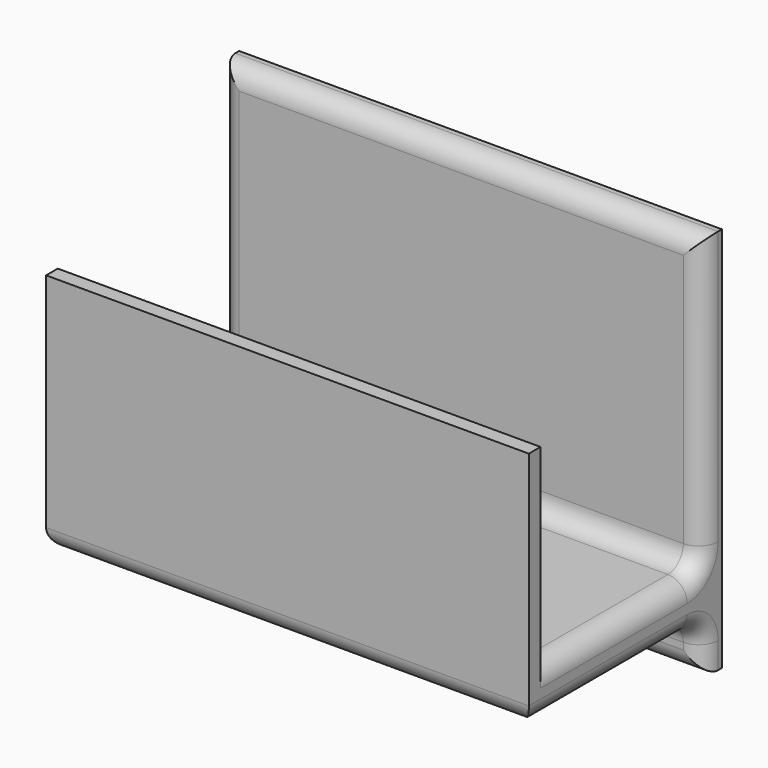
from build123d import *

# Parameters (mm, degrees)
F0_W     = 127
F0_H     = 12.7
F1_DEPTH = 63.5
F0_H_2   = 76.9474954844
F0_H_3   = 11.9525045156
F2_DEPTH = 6.35
F3_W     = 127
F3_H     = 3.8452798724
F4_DEPTH = 50.8
F5_R     = 5.08


with BuildPart() as f1:
    # F0 (on Front) → F1 (new body)
    with BuildSketch(Plane.XZ):
        with Locations((7.5608139634, -7.8621631652)):
            Rectangle(F0_W, F0_H)
    extrude(amount=F1_DEPTH)

    # F0 (on Front) → F2 (join)
    with BuildSketch(Plane.XZ):
        with Locations((7.5608139634, 36.961584577)):
            Rectangle(F0_W, F0_H_2)
        with Locations((7.5608139634, -20.188415423)):
            Rectangle(F0_W, F0_H_3)
        with Locations((7.5608139634, -7.8621631652)):
            Rectangle(F0_W, F0_H)
    extrude(amount=F2_DEPTH)

    # F3 (on face) → F4 (join)
    with BuildSketch(Plane.XY.offset(-1.5121631652)):
        with Locations((7.5608139634, -61.5773600638)):
            Rectangle(F3_W, F3_H)
    extrude(amount=F4_DEPTH)

    # F5
    f5_edges = [f1.edges().sort_by_distance(p)[0] for p in [
        (7.560814, -63.5, -14.212163),
        (71.060814, -34.925, -14.212163),
        (7.560814, -6.35, -26.164668),
        (-55.939186, -6.35, -20.188415),
        (-55.939186, -34.925, -14.212163),
        (71.060814, -6.35, -20.188415),
        (7.560814, -6.35, -14.212163),
        (-55.939186, -6.35, 36.961585),
        (7.560814, -6.35, -1.512163),
        (7.560814, -6.35, 75.435332),
        (71.060814, -33.00236, -1.512163),
        (71.060814, -6.35, 36.961585),
        (-55.939186, -33.00236, -1.512163),
    ]]
    fillet(f5_edges, radius=F5_R)


solid = f1.part
